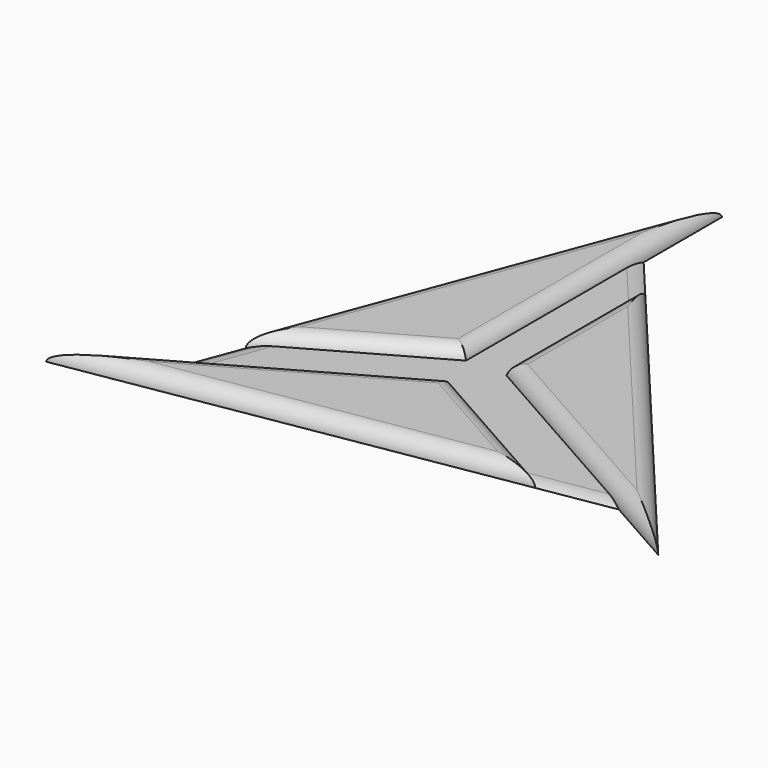
from build123d import *

# Parameters (mm, degrees)
F1_DEPTH     = 1.3
F2_R         = 1.29999
F2_2_R       = 1.29999
F2_3_R       = 1.29999
F4_DEPTH     = 0.3
F5_T4_DEPTH  = 14.2239553164
F5_T9_DEPTH  = 50.4507657891
F5_T14_DEPTH = 14.5398031116
F5_T19_DEPTH = 49.459435346
F5_T24_DEPTH = 13.2114658899
F5_T29_DEPTH = 50.9943998556
F5_T35_DEPTH = 14.2239553164
F5_T39_DEPTH = 50.4507657891
F5_T46_DEPTH = 14.5398031116
F5_T50_DEPTH = 49.459435346
F5_T57_DEPTH = 50.9943998556
F5_T61_DEPTH = 13.2114658899


# Not quite as in the source:
# - a fillet or chamfer that OpenCascade refuses, or shapes differently, is made with other operations: its cross-section is extruded or revolved along the edge and cut away or added
# - a fillet or chamfer is up to 0.001 mm smaller than in the source, because OpenCascade refuses the exact size


with BuildPart() as f1:
    # F0 (on Top) → F1 (new body)
    with BuildSketch(Plane.XY):
        Polygon((-24.0248936415, 49.8194298056), (-37.3686429682, 14.1594352904), (-24.0248936415, 21.7105125955), align=None)
    extrude(amount=F1_DEPTH)

    # F2 (radius 1.3 in the source; OpenCascade refuses exactly that, so slightly less here)
    f2_edges = [f1.edges().sort_by_distance(p)[0] for p in [
        (-30.696768, 31.989433, 1.3),
        (-30.696768, 17.934974, 1.3),
        (-24.024894, 35.764971, 1.3),
    ]]
    fillet(f2_edges, radius=F2_R)


with BuildPart() as f1b:
    # F0 (on Top) → F1, piece 2 (new body)
    with BuildSketch(Plane.XY):
        Polygon((-20.5248936415, 37.0426492555), (-20.5248936415, 21.7105125955), (3.9386467909, 7.8668708695), align=None)
    extrude(amount=F1_DEPTH)

    # F2#2 (radius 1.3 in the source; OpenCascade refuses exactly that, so slightly less here)
    f2_2_edges = [f1b.edges().sort_by_distance(p)[0] for p in [
        (-8.293123, 22.45476, 1.3),
        (-20.524894, 29.376581, 1.3),
        (-8.293123, 14.788692, 1.3),
    ]]
    fillet(f2_2_edges, radius=F2_2_R)


with BuildPart() as f1c:
    # F0 (on Top) → F1, piece 3 (new body)
    with BuildSketch(Plane.XY):
        Polygon((-22.2747167061, 17.947387251), (-46.8371441831, 4.0477864614), (-8.874694457, 10.3699137332), align=None)
    extrude(amount=F1_DEPTH)

    # F2#3 (radius 1.3 in the source; OpenCascade refuses exactly that, so slightly less here)
    f2_3_edges = [f1c.edges().sort_by_distance(p)[0] for p in [
        (-15.574706, 14.15865, 1.3),
        (-34.55593, 10.997587, 1.3),
        (-27.855919, 7.20885, 1.3),
    ]]
    fillet(f2_3_edges, radius=F2_3_R)


with BuildPart() as f4:
    # F3 (on face) → F4 (new body)
    with BuildSketch(Plane(origin=(0, 0, 0), x_dir=(1, 0, 0), z_dir=(0, 0, -1))):
        Polygon((-39.6251897876, -8.1290127133), (-24.0248936415, -49.8194298056), (-24.0248936415, -41.2167977375), (-20.5247644335, -37.0424725115), (3.9387424476, -7.8667970374), (-2.3921415244, -11.4494320516), (-8.8744852692, -10.3698913008), (-46.8372628093, -4.0477388538), align=None)
    extrude(amount=-F4_DEPTH)

    # F5: fillet of radius 2.5 on 6 edges, made by hand


with BuildPart() as f5_tool2:
    # F5_s3 → F5_t4 (new body)
    with BuildSketch(Plane(origin=(-36.3250135829, -20.5561324652, 0), x_dir=(0, 0, 1), z_dir=(0.8703102173, 0.4925039346, 0))):
        with BuildLine():
            ThreePointArc((0.3, -25.4028904918), (0.2238399287, -26.0152629275), (0, -26.5903247005))
            Line((0, -26.5903247005), (0.044, -26.6140733847))
            ThreePointArc((0.044, -26.6140733847), (0.15, -26.6403247005), (0.3, -26.6403247005))
            Line((0.3, -26.6403247005), (0.35, -26.5903247005))
            Line((0.35, -26.5903247005), (0.35, -25.4028904918))
            Line((0.35, -25.4028904918), (0.3, -25.4028904918))
        make_face()
    extrude(amount=F5_T4_DEPTH)

    split(bisect_by=Plane(origin=(-37.4265173045, 14.0047712254, 0), x_dir=(0, 0, 1), z_dir=(-0.9365771812, 0.3504613868, 0)), keep=Keep.TOP)


with BuildPart() as f4_1:
    add(f4.part)

    # F5_t1: cut F5_tool2
    add(f5_tool2.part, mode=Mode.SUBTRACT)


with BuildPart() as f5_tool7:
    # F5_s8 → F5_t9 (new body)
    with BuildSketch(Plane(origin=(-3.2390470819, -8.6560679722, 0), x_dir=(0, 0, 1), z_dir=(0.3504613868, 0.9365771812, 0))):
        with BuildLine():
            ThreePointArc((0.3, -38.7735194163), (0.2238399287, -39.385891852), (0, -39.960953625))
            Line((0, -39.960953625), (0.044, -39.9847023092))
            ThreePointArc((0.044, -39.9847023092), (0.15, -40.010953625), (0.3, -40.010953625))
            Line((0.3, -40.010953625), (0.35, -39.960953625))
            Line((0.35, -39.960953625), (0.35, -38.7735194163))
            Line((0.35, -38.7735194163), (0.3, -38.7735194163))
        make_face()
    extrude(amount=F5_T9_DEPTH)

    split(bisect_by=Plane(origin=(-13.095839537, 23.1418312694, 0), x_dir=(0, 0, 1), z_dir=(-0.4925039346, 0.8703102173, 0)), keep=Keep.TOP)


with BuildPart() as f4_2:
    add(f4_1.part)

    # F5_t6: cut F5_tool7
    add(f5_tool7.part, mode=Mode.SUBTRACT)


with BuildPart() as f5_tool12:
    # F5_s13 → F5_t14 (new body)
    with BuildSketch(Plane.XZ.offset(-52.7880153273)):
        with BuildLine():
            ThreePointArc((-25.2123278502, 0.3), (-24.5999554145, 0.2238399287), (-24.0248936415, 0))
            Line((-24.0248936415, 0), (-24.0011449573, 0.044))
            ThreePointArc((-24.0011449573, 0.044), (-23.9748936415, 0.15), (-23.9748936415, 0.3))
            Line((-23.9748936415, 0.3), (-24.0248936415, 0.35))
            Line((-24.0248936415, 0.35), (-25.2123278502, 0.35))
            Line((-25.2123278502, 0.35), (-25.2123278502, 0.3))
        make_face()
    extrude(amount=F5_T14_DEPTH)

    split(bisect_by=Plane(origin=(6.1858887221, 5.1868047221, 0), x_dir=(0, 0, 1), z_dir=(0.7662744858, 0.6425133558, 0)), keep=Keep.TOP)


with BuildPart() as f4_3:
    add(f4_2.part)

    # F5_t11: cut F5_tool12
    add(f5_tool12.part, mode=Mode.SUBTRACT)


with BuildPart() as f5_tool17:
    # F5_s18 → F5_t19 (new body)
    with BuildSketch(Plane(origin=(-32.1181382092, 38.3047443597, 0), x_dir=(0, 0, 1), z_dir=(0.6425133558, -0.7662744858, 0))):
        with BuildLine():
            ThreePointArc((0.3, -6.8852457991), (0.2238399287, -7.4976182348), (0, -8.0726800078))
            Line((0, -8.0726800078), (0.044, -8.0964286919))
            ThreePointArc((0.044, -8.0964286919), (0.15, -8.1226800078), (0.3, -8.1226800078))
            Line((0.3, -8.1226800078), (0.35, -8.0726800078))
            Line((0.35, -8.0726800078), (0.35, -6.8852457991))
            Line((0.35, -6.8852457991), (0.3, -6.8852457991))
        make_face()
    extrude(amount=F5_T19_DEPTH)

    split(bisect_by=Plane.YZ.offset(-24.0248936415), keep=Keep.TOP)


with BuildPart() as f4_4:
    add(f4_3.part)

    # F5_t16: cut F5_tool17
    add(f5_tool17.part, mode=Mode.SUBTRACT)


with BuildPart() as f5_tool22:
    # F5_s23 → F5_t24 (new body)
    with BuildSketch(Plane(origin=(2.194973472, -1.2421312491, 0), x_dir=(0, 0, 1), z_dir=(-0.8703089586, 0.492506159, 0))):
        with BuildLine():
            ThreePointArc((0.3, 9.9738330597), (0.2238399287, 9.361460624), (0, 8.786398851))
            Line((0, 8.786398851), (0.044, 8.7626501668))
            ThreePointArc((0.044, 8.7626501668), (0.15, 8.736398851), (0.3, 8.736398851))
            Line((0.3, 8.736398851), (0.35, 8.786398851))
            Line((0.35, 8.786398851), (0.35, 9.9738330597))
            Line((0.35, 9.9738330597), (0.3, 9.9738330597))
        make_face()
    extrude(amount=F5_T24_DEPTH)

    split(bisect_by=Plane(origin=(-1.9198365379, 11.5280876274, 0), x_dir=(0, 0, 1), z_dir=(0.1642731564, -0.9864148874, 0)), keep=Keep.TOP)


with BuildPart() as f4_5:
    add(f4_4.part)

    # F5_t21: cut F5_tool22
    add(f5_tool22.part, mode=Mode.SUBTRACT)


with BuildPart() as f5_tool27:
    # F5_s28 → F5_t29 (new body)
    with BuildSketch(Plane(origin=(2.4559519667, 0.4090033381, 0), x_dir=(0, 0, 1), z_dir=(-0.9864148874, -0.1642731564, 0))):
        with BuildLine():
            ThreePointArc((0, 11.6868548668), (0.2238399287, 12.2619166398), (0.3, 12.8742890755))
            Line((0.3, 12.8742890755), (0.35, 12.8742890755))
            Line((0.35, 12.8742890755), (0.35, 11.6868548668))
            Line((0.35, 11.6868548668), (0.3, 11.6368548668))
            ThreePointArc((0.3, 11.6368548668), (0.15, 11.6368548668), (0.044, 11.6631061826))
            Line((0.044, 11.6631061826), (0, 11.6868548668))
        make_face()
    extrude(amount=F5_T29_DEPTH)

    split(bisect_by=Plane(origin=(4.3273555495, 7.6468816335, 0), x_dir=(0, 0, 1), z_dir=(-0.492506159, -0.8703089586, 0)), keep=Keep.TOP)


with BuildPart() as f4_6:
    add(f4_5.part)

    # F5_t26: cut F5_tool27
    add(f5_tool27.part, mode=Mode.SUBTRACT)


with BuildPart() as f5_tool33:
    # F5_s34 → F5_t35 (new body)
    with BuildSketch(Plane(origin=(-36.3250135829, -20.5561324652, 0), x_dir=(0, 0, 1), z_dir=(0.8703102173, 0.4925039346, 0))):
        with BuildLine():
            ThreePointArc((0.3, -25.4028904918), (0.2238399287, -26.0152629275), (0, -26.5903247005))
            Line((0, -26.5903247005), (0.044, -26.6140733847))
            ThreePointArc((0.044, -26.6140733847), (0.15, -26.6403247005), (0.3, -26.6403247005))
            Line((0.3, -26.6403247005), (0.35, -26.5903247005))
            Line((0.35, -26.5903247005), (0.35, -25.4028904918))
            Line((0.35, -25.4028904918), (0.3, -25.4028904918))
        make_face()
    extrude(amount=F5_T35_DEPTH)

    split(bisect_by=Plane(origin=(-37.4265173045, 14.0047712254, 0), x_dir=(0, 0, 1), z_dir=(0.9365771812, -0.3504613868, 0)), keep=Keep.TOP)


with BuildPart() as f5_tool37:
    # F5_s38 → F5_t39 (new body)
    with BuildSketch(Plane(origin=(-3.2390470819, -8.6560679722, 0), x_dir=(0, 0, 1), z_dir=(0.3504613868, 0.9365771812, 0))):
        with BuildLine():
            ThreePointArc((0.3, -38.7735194163), (0.2238399287, -39.385891852), (0, -39.960953625))
            Line((0, -39.960953625), (0.044, -39.9847023092))
            ThreePointArc((0.044, -39.9847023092), (0.15, -40.010953625), (0.3, -40.010953625))
            Line((0.3, -40.010953625), (0.35, -39.960953625))
            Line((0.35, -39.960953625), (0.35, -38.7735194163))
            Line((0.35, -38.7735194163), (0.3, -38.7735194163))
        make_face()
    extrude(amount=F5_T39_DEPTH)

    split(bisect_by=Plane(origin=(-13.095839537, 23.1418312694, 0), x_dir=(0, 0, 1), z_dir=(0.4925039346, -0.8703102173, 0)), keep=Keep.TOP)


with BuildPart() as f5_tool33_1:
    add(f5_tool33.part)

    # F5_t41: intersect F5_tool37
    add(f5_tool37.part, mode=Mode.INTERSECT)


with BuildPart() as f4_7:
    add(f4_6.part)

    # F5_t31: cut F5_tool33
    add(f5_tool33_1.part, mode=Mode.SUBTRACT)


with BuildPart() as f5_tool44:
    # F5_s45 → F5_t46 (new body)
    with BuildSketch(Plane.XZ.offset(-52.7880153273)):
        with BuildLine():
            ThreePointArc((-25.2123278502, 0.3), (-24.5999554145, 0.2238399287), (-24.0248936415, 0))
            Line((-24.0248936415, 0), (-24.0011449573, 0.044))
            ThreePointArc((-24.0011449573, 0.044), (-23.9748936415, 0.15), (-23.9748936415, 0.3))
            Line((-23.9748936415, 0.3), (-24.0248936415, 0.35))
            Line((-24.0248936415, 0.35), (-25.2123278502, 0.35))
            Line((-25.2123278502, 0.35), (-25.2123278502, 0.3))
        make_face()
    extrude(amount=F5_T46_DEPTH)

    split(bisect_by=Plane(origin=(6.1858887221, 5.1868047221, 0), x_dir=(0, 0, 1), z_dir=(-0.7662744858, -0.6425133558, 0)), keep=Keep.TOP)


with BuildPart() as f5_tool48:
    # F5_s49 → F5_t50 (new body)
    with BuildSketch(Plane(origin=(-32.1181382092, 38.3047443597, 0), x_dir=(0, 0, 1), z_dir=(0.6425133558, -0.7662744858, 0))):
        with BuildLine():
            ThreePointArc((0.3, -6.8852457991), (0.2238399287, -7.4976182348), (0, -8.0726800078))
            Line((0, -8.0726800078), (0.044, -8.0964286919))
            ThreePointArc((0.044, -8.0964286919), (0.15, -8.1226800078), (0.3, -8.1226800078))
            Line((0.3, -8.1226800078), (0.35, -8.0726800078))
            Line((0.35, -8.0726800078), (0.35, -6.8852457991))
            Line((0.35, -6.8852457991), (0.3, -6.8852457991))
        make_face()
    extrude(amount=F5_T50_DEPTH)

    split(bisect_by=Plane.YZ.offset(-24.0248936415), keep=Keep.BOTTOM)


with BuildPart() as f5_tool44_1:
    add(f5_tool44.part)

    # F5_t52: intersect F5_tool48
    add(f5_tool48.part, mode=Mode.INTERSECT)


with BuildPart() as f4_8:
    add(f4_7.part)

    # F5_t42: cut F5_tool44
    add(f5_tool44_1.part, mode=Mode.SUBTRACT)


with BuildPart() as f5_tool55:
    # F5_s56 → F5_t57 (new body)
    with BuildSketch(Plane(origin=(2.4559519667, 0.4090033381, 0), x_dir=(0, 0, 1), z_dir=(-0.9864148874, -0.1642731564, 0))):
        with BuildLine():
            ThreePointArc((0, 11.6868548668), (0.2238399287, 12.2619166398), (0.3, 12.8742890755))
            Line((0.3, 12.8742890755), (0.35, 12.8742890755))
            Line((0.35, 12.8742890755), (0.35, 11.6868548668))
            Line((0.35, 11.6868548668), (0.3, 11.6368548668))
            ThreePointArc((0.3, 11.6368548668), (0.15, 11.6368548668), (0.044, 11.6631061826))
            Line((0.044, 11.6631061826), (0, 11.6868548668))
        make_face()
    extrude(amount=F5_T57_DEPTH)

    split(bisect_by=Plane(origin=(4.3273555495, 7.6468816335, 0), x_dir=(0, 0, 1), z_dir=(0.492506159, 0.8703089586, 0)), keep=Keep.TOP)


with BuildPart() as f5_tool59:
    # F5_s60 → F5_t61 (new body)
    with BuildSketch(Plane(origin=(2.194973472, -1.2421312491, 0), x_dir=(0, 0, 1), z_dir=(-0.8703089586, 0.492506159, 0))):
        with BuildLine():
            ThreePointArc((0.3, 9.9738330597), (0.2238399287, 9.361460624), (0, 8.786398851))
            Line((0, 8.786398851), (0.044, 8.7626501668))
            ThreePointArc((0.044, 8.7626501668), (0.15, 8.736398851), (0.3, 8.736398851))
            Line((0.3, 8.736398851), (0.35, 8.786398851))
            Line((0.35, 8.786398851), (0.35, 9.9738330597))
            Line((0.35, 9.9738330597), (0.3, 9.9738330597))
        make_face()
    extrude(amount=F5_T61_DEPTH)

    split(bisect_by=Plane(origin=(-1.9198365379, 11.5280876274, 0), x_dir=(0, 0, 1), z_dir=(-0.1642731564, 0.9864148874, 0)), keep=Keep.TOP)


with BuildPart() as f5_tool55_1:
    add(f5_tool55.part)

    # F5_t63: intersect F5_tool59
    add(f5_tool59.part, mode=Mode.INTERSECT)


with BuildPart() as f4_9:
    add(f4_8.part)

    # F5_t53: cut F5_tool55
    add(f5_tool55_1.part, mode=Mode.SUBTRACT)


solid = Compound([f1.part, f1b.part, f1c.part, f4_9.part])
